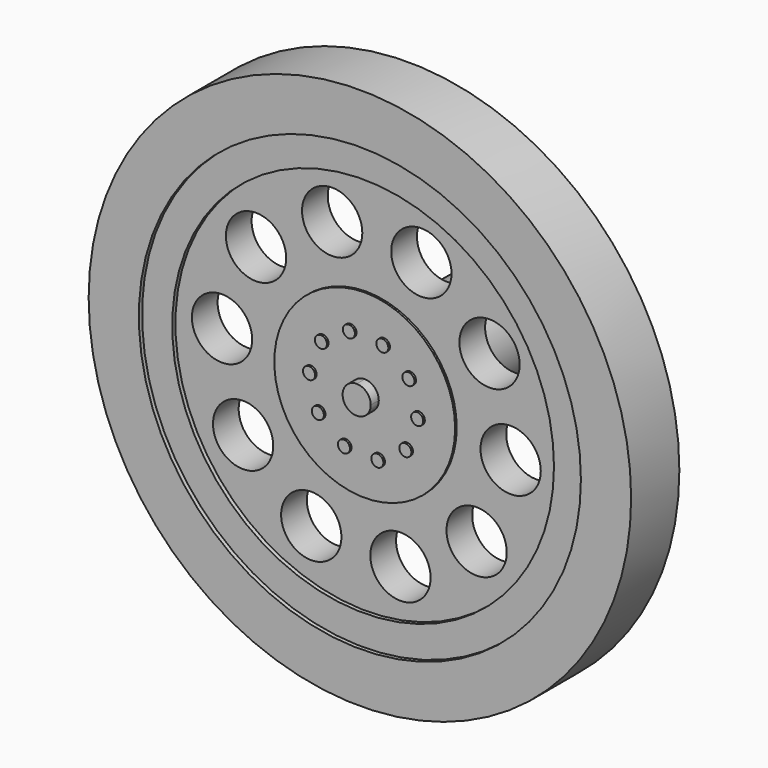
from build123d import *

# Parameters (mm, degrees)
F0_R      = 17.145
F0_R_2    = 13.97
F1_DEPTH  = 0.762
F0_R_3    = 12.065
F2_DEPTH  = 0.508
F3_DEPTH  = 0.254
F0_R_4    = 0.381
F5_DEPTH  = 0.381
F6_DEPTH  = 0.508
F7_DEPTH  = 1.016
F8_R      = 1.905
F9_DEPTH  = 25.4
F10_DEPTH = 3.048
F11_R     = 3.048
F11_R_2   = 1.905
F12_DEPTH = 8.128
F13_R     = 13.97
F13_R_2   = 12.065
F14_DEPTH = 0.762
F15_DEPTH = 1.27


# Not quite as in the source:
# - the program builds the solid bodies; features that only make, move or delete a surface that nothing else refers to are left out


with BuildPart() as f1:
    # F0 (on Front) → F1 (new body)
    with BuildSketch(Plane.XZ):
        Circle(F0_R)
        Circle(F0_R_2, mode=Mode.SUBTRACT)
    extrude(amount=F1_DEPTH)

    # F0 (on Front) → F2 (join)
    with BuildSketch(Plane.XZ):
        Circle(F0_R_2)
        Circle(F0_R_3, mode=Mode.SUBTRACT)
    extrude(amount=F2_DEPTH)

    # F0 (on Front) → F3 (join)
    with BuildSketch(Plane.XZ):
        Circle(F0_R_3)
        with BuildLine():
            ThreePointArc((0, 5.715), (4.0411152545, 4.0411152545), (5.715, 0))
            ThreePointArc((5.715, 0), (-4.0411152545, -4.0411152545), (0, 5.715))
        make_face(mode=Mode.SUBTRACT)
    extrude(amount=F3_DEPTH)

    # F0 (on Front) → F5 (join)
    with BuildSketch(Plane.XZ):
        with BuildLine():
            ThreePointArc((0, 5.715), (-4.0411152545, -4.0411152545), (5.715, 0))
            ThreePointArc((5.715, 0), (4.0411152545, 4.0411152545), (0, 5.715))
        make_face()
        with Locations((-1.2134722805, -3.1998572434)):
            Circle(F0_R_4, mode=Mode.SUBTRACT)
        with Locations((-2.8625485942, -1.8754777789)):
            Circle(F0_R_4, mode=Mode.SUBTRACT)
        with Locations((0.8991092, -3.302)):
            Circle(F0_R_4, mode=Mode.SUBTRACT)
        with Locations((2.6682615257, -2.1428909875)):
            Circle(F0_R_4, mode=Mode.SUBTRACT)
        with Locations((3.4182286394, -0.1652704519)):
            Circle(F0_R_4, mode=Mode.SUBTRACT)
        with Locations((-3.4182286394, 0.1652704519)):
            Circle(F0_R_4, mode=Mode.SUBTRACT)
        with Locations((-2.6682615257, 2.1428909875)):
            Circle(F0_R_4, mode=Mode.SUBTRACT)
        with Locations((-0.8991092, 3.302)):
            Circle(F0_R_4, mode=Mode.SUBTRACT)
        with BuildLine():
            ThreePointArc((0.889, 0), (-0.6286179285, -0.6286179285), (0, 0.889))
            ThreePointArc((0, 0.889), (0.6286179285, 0.6286179285), (0.889, 0))
        make_face(mode=Mode.SUBTRACT)
        with Locations((2.8625485942, 1.8754777789)):
            Circle(F0_R_4, mode=Mode.SUBTRACT)
        with BuildLine():
            ThreePointArc((1.5944722805, 3.1998572434), (1.161927001, 2.8223601121), (0.8464193452, 3.302))
            ThreePointArc((0.8464193452, 3.302), (1.2650175599, 3.5773543747), (1.5944722805, 3.1998572434))
        make_face(mode=Mode.SUBTRACT)
    extrude(amount=F5_DEPTH)

    # F0 (on Front) → F6 (join)
    with BuildSketch(Plane.XZ):
        with Locations((-0.8991092, 3.302)):
            Circle(F0_R_4)
        with BuildLine():
            ThreePointArc((1.5944722805, 3.1998572434), (1.2650175599, 3.5773543747), (0.8464193452, 3.302))
            ThreePointArc((0.8464193452, 3.302), (1.161927001, 2.8223601121), (1.5944722805, 3.1998572434))
        make_face()
        with Locations((-2.6682615257, 2.1428909875)):
            Circle(F0_R_4)
        with Locations((2.8625485942, 1.8754777789)):
            Circle(F0_R_4)
        with Locations((3.4182286394, -0.1652704519)):
            Circle(F0_R_4)
        with Locations((-1.2134722805, -3.1998572434)):
            Circle(F0_R_4)
        with Locations((-2.8625485942, -1.8754777789)):
            Circle(F0_R_4)
        with Locations((-3.4182286394, 0.1652704519)):
            Circle(F0_R_4)
        with Locations((2.6682615257, -2.1428909875)):
            Circle(F0_R_4)
        with Locations((0.8991092, -3.302)):
            Circle(F0_R_4)
    extrude(amount=F6_DEPTH)

    # F0 (on Front) → F7 (join)
    with BuildSketch(Plane.XZ):
        with BuildLine():
            ThreePointArc((0.889, 0), (0.6286179285, 0.6286179285), (0, 0.889))
            ThreePointArc((0, 0.889), (-0.6286179285, -0.6286179285), (0.889, 0))
        make_face()
    extrude(amount=F7_DEPTH)

    # F8 (on face) → F9 (cut)
    with BuildSketch(Plane.XZ.offset(0.254)):
        with Locations((-2.1587662638, 8.89)):
            Circle(F8_R)
        with Locations((-6.9718894872, 5.923270107)):
            Circle(F8_R)
        with Locations((-9.1219878923, 0.6940523577)):
            Circle(F8_R)
        with Locations((-7.7877969675, -4.8002698023)):
            Circle(F8_R)
        with Locations((-3.4789322986, -8.461052053)):
            Circle(F8_R)
        with Locations((2.1587662638, -8.89)):
            Circle(F8_R)
        with Locations((6.9718894872, -5.923270107)):
            Circle(F8_R)
        with Locations((9.1219878923, -0.6940523577)):
            Circle(F8_R)
        with Locations((7.7877969675, 4.8002698023)):
            Circle(F8_R)
        with Locations((3.4789322986, 8.461052053)):
            Circle(F8_R)
    extrude(amount=-F9_DEPTH, mode=Mode.SUBTRACT)

    # F10 (add): a face of the model
    f10_faces = [f1.faces().sort_by_distance(p)[0] for p in [
        (0, 0, 0),
    ]]
    extrude(f10_faces, amount=F10_DEPTH)

    # F11 (on face) → F12 (join)
    with BuildSketch(Plane(origin=(0, 3.048, 0), x_dir=(-1, 0, 0), z_dir=(0, 1, 0))):
        Circle(F11_R)
        Circle(F11_R_2, mode=Mode.SUBTRACT)
    extrude(amount=F12_DEPTH)

    # F13 (on face) → F14 (cut)
    with BuildSketch(Plane(origin=(0, 3.048, 0), x_dir=(-1, 0, 0), z_dir=(0, 1, 0))):
        Circle(F13_R)
        Circle(F13_R_2, mode=Mode.SUBTRACT)
    extrude(amount=-F14_DEPTH, mode=Mode.SUBTRACT)

    # F15 (cut): a face of the model
    f15_faces = [f1.faces().sort_by_distance(p)[0] for p in [
        (11.7237502674, 3.048, 0),
    ]]
    extrude(f15_faces, amount=-F15_DEPTH, mode=Mode.SUBTRACT)


solid = f1.part
